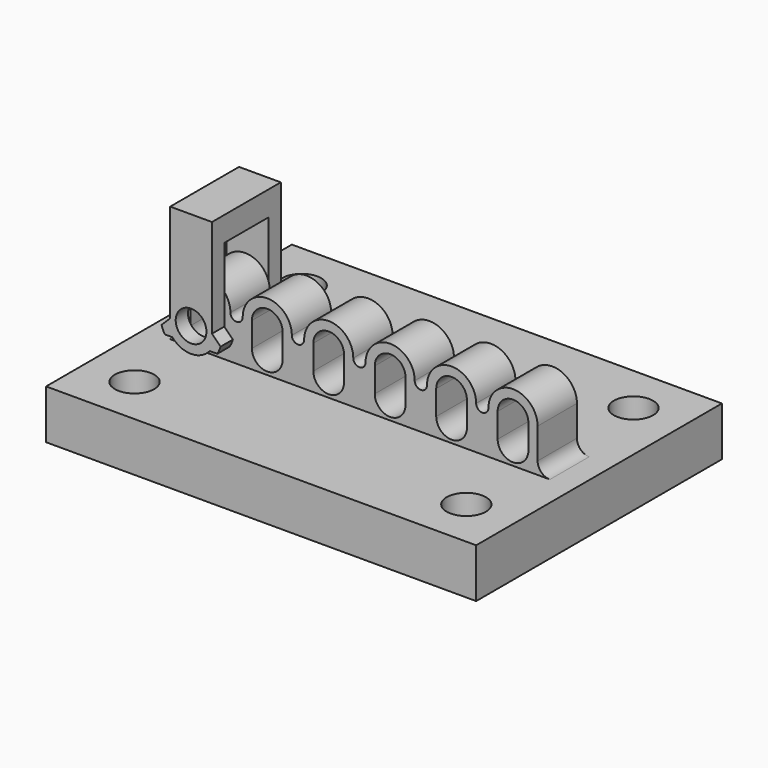
from build123d import *

# Parameters (mm, degrees)
F1_DEPTH      = 2
F2_W          = 35
F2_H          = 4
F3_DEPTH      = 10
F3_DEPTH_BACK = 15
F4_R          = 1.6
F5_DEPTH      = 6.5
F6_R          = 1.25
F7_DEPTH      = 3.5
F8_W          = 4.5
F8_H          = 8.2
F9_DEPTH      = 12.5


with BuildPart() as f1:
    # F0 (on Front) → F1 (new body, symmetric)
    with BuildSketch(Plane.XZ):
        with BuildLine():
            Line((-5, -2.5), (-5, -6.5))
            Line((-5, -6.5), (30, -6.5))
            Line((30, -6.5), (30, -2.5))
            Line((30, -2.5), (28, -2.5))
            ThreePointArc((28, -2.5), (27.2928932188, -2.2071067812), (27, -1.5))
            Line((27, -1.5), (27, 1))
            ThreePointArc((27, 1), (25, 3), (23, 1))
            ThreePointArc((23, 1), (22.5, 0.5), (22, 1))
            ThreePointArc((22, 1), (20, 3), (18, 1))
            ThreePointArc((18, 1), (17.5, 0.5), (17, 1))
            ThreePointArc((17, 1), (15, 3), (13, 1))
            ThreePointArc((13, 1), (12.5, 0.5), (12, 1))
            ThreePointArc((12, 1), (10, 3), (8, 1))
            ThreePointArc((8, 1), (7.5, 0.5), (7, 1))
            ThreePointArc((7, 1), (5, 3), (3, 1))
            ThreePointArc((3, 1), (2.5, 0.5), (2, 1))
            ThreePointArc((2, 1), (0, 3), (-2, 1))
            Line((-2, 1), (-2, -1.5))
            ThreePointArc((-2, -1.5), (-2.2928932188, -2.2071067812), (-3, -2.5))
            Line((-3, -2.5), (-5, -2.5))
        make_face()
        with BuildLine():
            Line((-1.25, -1), (-1.25, 1))
            ThreePointArc((-1.25, 1), (0, 2.25), (1.25, 1))
            Line((1.25, 1), (1.25, -1))
            ThreePointArc((1.25, -1), (0, -2.25), (-1.25, -1))
        make_face(mode=Mode.SUBTRACT)
        with BuildLine():
            ThreePointArc((6.25, -1), (5, -2.25), (3.75, -1))
            Line((3.75, -1), (3.75, 1))
            ThreePointArc((3.75, 1), (5, 2.25), (6.25, 1))
            Line((6.25, 1), (6.25, -1))
        make_face(mode=Mode.SUBTRACT)
        with BuildLine():
            ThreePointArc((11.25, -1), (10, -2.25), (8.75, -1))
            Line((8.75, -1), (8.75, 1))
            ThreePointArc((8.75, 1), (10, 2.25), (11.25, 1))
            Line((11.25, 1), (11.25, -1))
        make_face(mode=Mode.SUBTRACT)
        with BuildLine():
            ThreePointArc((16.25, -1), (15, -2.25), (13.75, -1))
            Line((13.75, -1), (13.75, 1))
            ThreePointArc((13.75, 1), (15, 2.25), (16.25, 1))
            Line((16.25, 1), (16.25, -1))
        make_face(mode=Mode.SUBTRACT)
        with BuildLine():
            ThreePointArc((21.25, -1), (20, -2.25), (18.75, -1))
            Line((18.75, -1), (18.75, 1))
            ThreePointArc((18.75, 1), (20, 2.25), (21.25, 1))
            Line((21.25, 1), (21.25, -1))
        make_face(mode=Mode.SUBTRACT)
        with BuildLine():
            ThreePointArc((26.25, -1), (25, -2.25), (23.75, -1))
            Line((23.75, -1), (23.75, 1))
            ThreePointArc((23.75, 1), (25, 2.25), (26.25, 1))
            Line((26.25, 1), (26.25, -1))
        make_face(mode=Mode.SUBTRACT)
    extrude(amount=F1_DEPTH, both=True)

    # F2 (on face) → F3 (join, two sides)
    with BuildSketch(Plane.XZ.offset(2)) as f3_sk:
        with Locations((12.5, -4.5)):
            Rectangle(F2_W, F2_H)
    extrude(amount=F3_DEPTH)
    extrude(f3_sk.sketch, amount=-F3_DEPTH_BACK)

    # F4 (on Top) → F5 (cut, through all)
    with BuildSketch(Plane.XY):
        with Locations((-1, 9)):
            Circle(F4_R)
        with Locations((26, 9)):
            Circle(F4_R)
        with Locations((26, -8)):
            Circle(F4_R)
        with Locations((-1, -8)):
            Circle(F4_R)
    extrude(amount=-F5_DEPTH, mode=Mode.SUBTRACT)


with BuildPart() as f7:
    # F6 (on Front) → F7 (new body, symmetric)
    with BuildSketch(Plane.XZ):
        with BuildLine():
            Line((-2.1354156504, -1.3), (-1.5198684154, -1.3))
            ThreePointArc((-1.5198684154, -1.3), (0, -2), (1.5198684154, -1.3))
            Line((1.5198684154, -1.3), (2.1354156504, -1.3))
            ThreePointArc((2.1354156504, -1.3), (2.2874655802, -1.0087126546), (2.4, -0.7))
            Line((2.4, -0.7), (1.7, 0))
            Line((1.7, 0), (1.7, 8))
            Line((1.7, 8), (-1.7, 8))
            Line((-1.7, 8), (-1.7, 0))
            Line((-1.7, 0), (-2.4, -0.7))
            ThreePointArc((-2.4, -0.7), (-2.2874655802, -1.0087126546), (-2.1354156504, -1.3))
        make_face()
        Circle(F6_R, mode=Mode.SUBTRACT)
    extrude(amount=F7_DEPTH, both=True)

    # F8 (on Right) → F9 (cut, symmetric)
    with BuildSketch(Plane.YZ):
        with Locations((0, 1.9)):
            Rectangle(F8_W, F8_H)
    extrude(amount=F9_DEPTH, both=True, mode=Mode.SUBTRACT)


solid = Compound([f1.part, f7.part])
